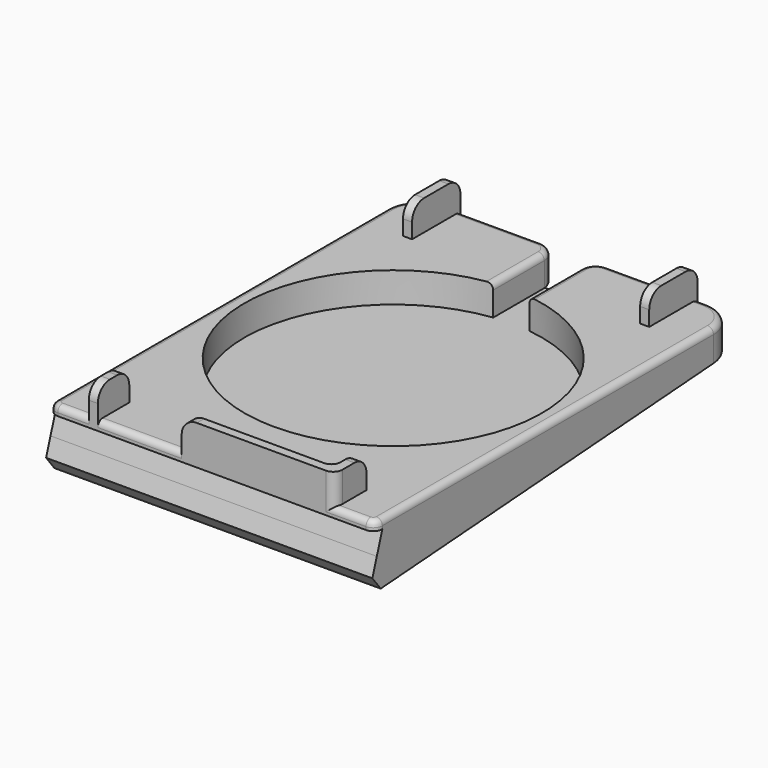
from build123d import *

# Parameters (mm, degrees)
F1_DEPTH      = 10
F3_DEPTH      = 10
F5_DEPTH      = 112.1
F6_DEPTH      = 112.8
F7_DEPTH      = 108
F2_W          = 3
F2_H          = 20
F2_H_2        = 13
F8_DEPTH      = 10
F9_T4_DEPTH   = 34.3846000786
F9_T9_DEPTH   = 34.3846000786
F10_R         = 10
F11_R         = 5
F12_R         = 2
F13_R         = 3
F14_T2_ANGLE  = 90
F14_T4_ANGLE  = 90
F14_T8_DEPTH  = 10.5
F14_T13_DEPTH = 10.5
F15_SIZE      = 5


# Not quite as in the source:
# - a fillet or chamfer that OpenCascade refuses, or shapes differently, is made with other operations: its cross-section is extruded or revolved along the edge and cut away or added
# - a feature names something its author has since deleted; it is built from what else it names


with BuildPart() as f1:
    # F0 (on Top) → F1 (new body)
    with BuildSketch(Plane.XY):
        with BuildLine():
            Line((17.5125259459, 108.1324160099), (-30.4874740541, 108.1324160099))
            Line((-30.4874740541, 108.1324160099), (-30.4874740541, -41.8675839901))
            Line((-30.4874740541, -41.8675839901), (77.5125259459, -41.8675839901))
            Line((77.5125259459, -41.8675839901), (77.5125259459, 108.1324160099))
            Line((77.5125259459, 108.1324160099), (29.5125259459, 108.1324160099))
            Line((29.5125259459, 108.1324160099), (29.5125259459, 82.0155675041))
            ThreePointArc((29.5125259459, 82.0155675041), (23.5125259459, -16.1175839901), (17.5125259459, 82.0155675041))
            Line((17.5125259459, 82.0155675041), (17.5125259459, 108.1324160099))
        make_face()
    extrude(amount=F1_DEPTH)

    # F2 (on face) → F3 (join)
    with BuildSketch(Plane.XY.offset(10)):
        Polygon((13.5125259459, -41.8675839901), (23.5125259459, -41.8675839901), (61.2625259459, -41.8675839901), (61.2625259459, -38.8675839901), (13.5125259459, -38.8675839901), align=None)
    extrude(amount=F3_DEPTH)

    # F4 (on face) → F5 (cut)
    with BuildSketch(Plane.YZ.offset(77.5125259459)):
        Polygon((-38.8675839901, 7), (-41.8675839901, 7), (-41.8675839901, 0), (-41.1420218637, 0), align=None)
    extrude(amount=-F5_DEPTH, mode=Mode.SUBTRACT)

    # F4 (on face) → F6 (cut)
    with BuildSketch(Plane.YZ.offset(77.5125259459)):
        Polygon((108.1324160099, 0), (108.1324160099, 0.6153999214), (103.3824160099, 0), align=None)
    extrude(amount=-F6_DEPTH, mode=Mode.SUBTRACT)

    # F4 (on face) → F7 (join)
    with BuildSketch(Plane.YZ.offset(77.5125259459)):
        Polygon((-38.8675839901, 0), (-41.1420218637, 0), (-44.5225949872, -10.4043342482), (103.3824160099, 0), (-36.5935839901, 0), align=None)
    extrude(amount=-F7_DEPTH)

    # F2 (on face) → F8 (join)
    with BuildSketch(Plane.XY.offset(10)):
        with Locations((-15.7374740541, 98.1324160099)):
            Rectangle(F2_W, F2_H)
        with Locations((62.7625259459, 98.1324160099)):
            Rectangle(F2_W, F2_H)
        with Locations((-15.7374740541, -35.3675839901)):
            Rectangle(F2_W, F2_H_2)
        Polygon((61.2625259459, -38.8675839901), (61.2625259459, -41.8675839901), (64.2625259459, -41.8675839901), (64.2625259459, -28.8675839901), (61.2625259459, -28.8675839901), align=None)
    extrude(amount=F8_DEPTH)

    # F9: fillet of radius 5 on 2 edges, made by hand


with BuildPart() as f9_tool2:
    # F9_s3 → F9_t4 (new body)
    with BuildSketch(Plane.XY.offset(-11.8846000786)):
        with BuildLine():
            ThreePointArc((17.5125259459, 103.1324160099), (16.0480598518, 106.6679499158), (12.5125259459, 108.1324160099))
            Line((12.5125259459, 108.1324160099), (17.5125259459, 108.1324160099))
            Line((17.5125259459, 108.1324160099), (17.5125259459, 103.1324160099))
        make_face()
    extrude(amount=F9_T4_DEPTH)

    split(bisect_by=Plane.XY, keep=Keep.TOP)


with BuildPart() as f1_1:
    add(f1.part)

    # F9_t1: cut F9_tool2
    add(f9_tool2.part, mode=Mode.SUBTRACT)


with BuildPart() as f9_tool7:
    # F9_s8 → F9_t9 (new body)
    with BuildSketch(Plane.XY.offset(-11.8846000786)):
        with BuildLine():
            ThreePointArc((29.5125259459, 103.1324160099), (30.97699204, 106.6679499158), (34.5125259459, 108.1324160099))
            Line((34.5125259459, 108.1324160099), (29.5125259459, 108.1324160099))
            Line((29.5125259459, 108.1324160099), (29.5125259459, 103.1324160099))
        make_face()
    extrude(amount=F9_T9_DEPTH)

    split(bisect_by=Plane.XY, keep=Keep.TOP)


with BuildPart() as f1_2:
    add(f1_1.part)

    # F9_t6: cut F9_tool7
    add(f9_tool7.part, mode=Mode.SUBTRACT)

    # F10
    f10_edges = [f1_2.edges().sort_by_distance(p)[0] for p in [
        (77.512526, 108.132416, 5.3077),
        (-30.487474, 108.132416, 5.3077),
    ]]
    fillet(f10_edges, radius=F10_R)

    # F11
    f11_edges = [f1_2.edges().sort_by_distance(p)[0] for p in [
        (-15.737474, 88.132416, 20),
        (-15.737474, 108.132416, 20),
        (62.762526, 88.132416, 20),
        (62.762526, 108.132416, 20),
        (62.762526, -28.867584, 20),
        (-15.737474, -28.867584, 20),
        (-15.737474, -41.867584, 20),
        (13.512526, -40.367584, 20),
    ]]
    fillet(f11_edges, radius=F11_R)

    # F12
    f12_edges = [f1_2.edges().sort_by_distance(p)[0] for p in [
        (77.512526, 28.132416, 10),
        (-0.362474, -41.867584, 10),
        (70.887526, -41.867584, 10),
        (-23.862474, -41.867584, 10),
        (-30.487474, 28.132416, 10),
        (-27.558542, 105.203484, 10),
        (-18.862474, 108.132416, 10),
        (-0.862474, 108.132416, 10),
        (47.887526, 108.132416, 10),
        (74.583594, 105.203484, 10),
        (65.887526, 108.132416, 10),
        (30.976992, 106.66795, 10),
        (29.512526, 92.573992, 10),
        (17.512526, 92.573992, 10),
        (16.04806, 106.66795, 10),
    ]]
    fillet(f12_edges, radius=F12_R)

    # F13
    f13_edges = [f1_2.edges().sort_by_distance(p)[0] for p in [
        (64.262526, -41.867584, 15),
        (61.262526, -38.867584, 15),
    ]]
    fillet(f13_edges, radius=F13_R)

    # F14: fillet of radius 3 on 2 edges, made by hand

    # F14_s1 → F14_t2 (revolve, cut)
    with BuildSketch(Plane.XZ.offset(38.8675839901)):
        with BuildLine():
            ThreePointArc((-28.4874740541, 10), (-29.9016876165, 9.4142135624), (-30.4874740541, 8))
            Line((-30.4874740541, 8), (-30.4874740541, 10))
            Line((-30.4874740541, 10), (-28.4874740541, 10))
        make_face()
    revolve(axis=Axis((-27.4874740541, -38.8675839901, 10), (0, 0, 1)), revolution_arc=F14_T2_ANGLE, mode=Mode.SUBTRACT)

    # F14_s3 → F14_t4 (revolve, cut)
    with BuildSketch(Plane.YZ.offset(74.5125259459)):
        with BuildLine():
            ThreePointArc((-39.8675839901, 10), (-41.2817975525, 9.4142135624), (-41.8675839901, 8))
            Line((-41.8675839901, 8), (-41.8675839901, 10))
            Line((-41.8675839901, 10), (-39.8675839901, 10))
        make_face()
    revolve(axis=Axis((74.5125259459, -38.8675839901, 10), (0, 0, 1)), revolution_arc=F14_T4_ANGLE, mode=Mode.SUBTRACT)


with BuildPart() as f14_tool6:
    # F14_s7 → F14_t8 (new body)
    with BuildSketch(Plane.XY.offset(-0.5)):
        with BuildLine():
            ThreePointArc((74.5125259459, -41.8675839901), (76.6338462895, -40.9889043337), (77.5125259459, -38.8675839901))
            Line((77.5125259459, -38.8675839901), (77.5125259459, -41.8675839901))
            Line((77.5125259459, -41.8675839901), (74.5125259459, -41.8675839901))
        make_face()
    extrude(amount=F14_T8_DEPTH)

    split(bisect_by=Plane(origin=(0, -37.2133083672, 12.0913368505), x_dir=(1, 0, 0), z_dir=(0, -0.9510565163, 0.3090169944)), keep=Keep.TOP)


with BuildPart() as f1_3:
    add(f1_2.part)

    # F14_t5: cut F14_tool6
    add(f14_tool6.part, mode=Mode.SUBTRACT)


with BuildPart() as f14_tool11:
    # F14_s12 → F14_t13 (new body)
    with BuildSketch(Plane.XY.offset(-0.5)):
        with BuildLine():
            ThreePointArc((-27.4874740541, -41.8675839901), (-29.6087943977, -40.9889043337), (-30.4874740541, -38.8675839901))
            Line((-30.4874740541, -38.8675839901), (-30.4874740541, -41.8675839901))
            Line((-30.4874740541, -41.8675839901), (-27.4874740541, -41.8675839901))
        make_face()
    extrude(amount=F14_T13_DEPTH)

    split(bisect_by=Plane(origin=(0, -37.2133083672, 12.0913368505), x_dir=(1, 0, 0), z_dir=(0, -0.9510565163, 0.3090169944)), keep=Keep.TOP)


with BuildPart() as f1_4:
    add(f1_3.part)

    # F14_t10: cut F14_tool11
    add(f14_tool11.part, mode=Mode.SUBTRACT)

    # F15
    f15_edges = [f1_4.edges().sort_by_distance(p)[0] for p in [
        (23.512526, -44.522595, -10.404334),
    ]]
    chamfer(f15_edges, length=F15_SIZE)


solid = f1_4.part
